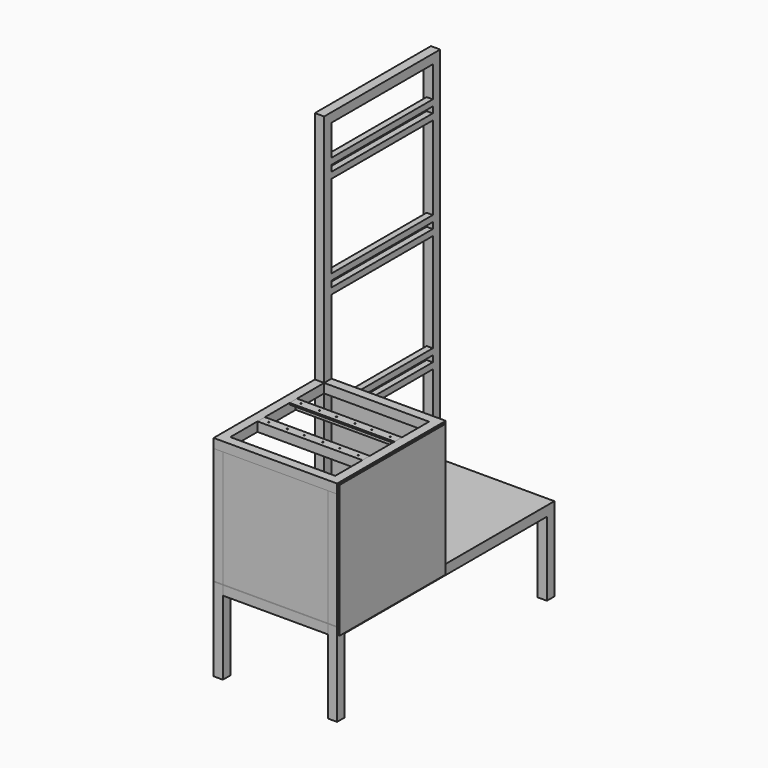
from build123d import *

# Parameters (mm, degrees)
F0_W          = 38.1
F0_H          = 38.1
F1_DEPTH      = 1117.6
F2_W          = 38.1
F2_H          = 38.1
F3_DEPTH      = 304.8
F3_DEPTH_BACK = 558.8
F4_W          = 38.1
F4_H          = 38.1
F5_DEPTH      = 304.8
F5_DEPTH_BACK = 1524
F6_W          = 38.1
F6_H          = 38.1
F7_DEPTH      = 1485.9
F8_W          = 38.1
F8_H          = 38.1
F9_DEPTH      = 431.8
F10_W         = 38.1
F10_H         = 38.1
F11_DEPTH     = 304.8
F12_W         = 38.1
F12_H         = 38.1
F13_DEPTH     = 520.7
F14_W         = 508
F14_H         = 558.8
F14_W_2       = 431.8
F14_H_2       = 482.6
F15_DEPTH     = 38.1
F16_W         = 38.1
F16_H         = 38.1
F17_DEPTH     = 431.8
F18_W         = 38.1
F18_H         = 38.1
F19_DEPTH     = 520.7
F21_DEPTH     = 431.8
F24_W         = 508
F24_H         = 1117.6
F25_DEPTH     = 2.54
F26_W         = 431.8
F26_H         = 482.6
F27_DEPTH     = 1.27
F28_W         = 431.8
F28_H         = 480.06
F29_DEPTH     = 1.27
F30_W         = 546.1
F30_H         = 546.1
F31_DEPTH     = 5.08
F32_W         = 25.4
F32_H         = 25.4
F33_DEPTH     = 520.7
F34_R         = 2.54
F35_DEPTH     = 6.35


with BuildPart() as f1:
    # F0 (on Front) → F1 (new body)
    with BuildSketch(Plane.XZ):
        Rectangle(F0_W, F0_H)
    extrude(amount=F1_DEPTH)

    # F4 (on face) → F5 (join, two sides)
    with BuildSketch(Plane(origin=(0, 0, -19.05), x_dir=(1, 0, 0), z_dir=(0, 0, -1))) as f5_sk:
        with Locations((0, 19.05)):
            Rectangle(F4_W, F4_H)
    extrude(amount=F5_DEPTH)
    extrude(f5_sk.sketch, amount=-F5_DEPTH_BACK)

    # F6 (on face) → F7 (join, through all)
    with BuildSketch(Plane.XY.offset(19.05)):
        with Locations((0, -577.85)):
            Rectangle(F6_W, F6_H)
    extrude(amount=F7_DEPTH)

    # F18 (on face) → F19 (join, through all)
    with BuildSketch(Plane.XZ.offset(38.1)):
        with Locations((0, 1485.9)):
            Rectangle(F18_W, F18_H)
    extrude(amount=F19_DEPTH)

    # F32 (on face) → F33 (join, through all)
    with BuildSketch(Plane(origin=(0, -558.8, 0), x_dir=(-1, 0, 0), z_dir=(0, 1, 0))):
        with Locations((-6.35, 425.45)):
            Rectangle(F32_W, F32_H)
        with Locations((-6.35, 908.05)):
            Rectangle(F32_W, F32_H)
        with Locations((-6.35, 1327.15)):
            Rectangle(F32_W, F32_H)
        with Locations((-6.35, 1276.35)):
            Rectangle(F32_W, F32_H)
        with Locations((-6.35, 857.25)):
            Rectangle(F32_W, F32_H)
        with Locations((-6.35, 374.65)):
            Rectangle(F32_W, F32_H)
    extrude(amount=F33_DEPTH)


with BuildPart() as f1b:
    # F0 (on Front) → F1, piece 2 (new body)
    with BuildSketch(Plane.XZ):
        with Locations((469.9, 0)):
            Rectangle(F0_W, F0_H)
    extrude(amount=F1_DEPTH)

    # F10 (on face) → F11 (join, through all)
    with BuildSketch(Plane(origin=(0, 0, -19.05), x_dir=(1, 0, 0), z_dir=(0, 0, -1))):
        with Locations((469.9, 19.05)):
            Rectangle(F10_W, F10_H)
    extrude(amount=F11_DEPTH)

    # F12 (on face) → F13 (join, through all)
    with BuildSketch(Plane.XY.offset(19.05)):
        with Locations((469.9, -577.85)):
            Rectangle(F12_W, F12_H)
    extrude(amount=F13_DEPTH)


with BuildPart() as f3:
    # F2 (on face) → F3 (new body, two sides)
    with BuildSketch(Plane(origin=(0, 0, -19.05), x_dir=(1, 0, 0), z_dir=(0, 0, -1))) as f3_sk:
        with Locations((469.9, 1098.55)):
            Rectangle(F2_W, F2_H)
    extrude(amount=F3_DEPTH)
    extrude(f3_sk.sketch, amount=-F3_DEPTH_BACK)


with BuildPart() as f3b:
    # F2 (on face) → F3, piece 2 (new body, two sides)
    with BuildSketch(Plane(origin=(0, 0, -19.05), x_dir=(1, 0, 0), z_dir=(0, 0, -1))) as f3_2_sk:
        with Locations((0, 1098.55)):
            Rectangle(F2_W, F2_H)
    extrude(amount=F3_DEPTH)
    extrude(f3_2_sk.sketch, amount=-F3_DEPTH_BACK)


with BuildPart() as f9:
    # F8 (on face) → F9 (new body, through all)
    with BuildSketch(Plane.YZ.offset(19.05)):
        with Locations((-1098.55, 0)):
            Rectangle(F8_W, F8_H)
    extrude(amount=F9_DEPTH)


with BuildPart() as f9b:
    # F8 (on face) → F9, piece 2 (new body, through all)
    with BuildSketch(Plane.YZ.offset(19.05)):
        with Locations((-19.05, 0)):
            Rectangle(F8_W, F8_H)
    extrude(amount=F9_DEPTH)


with BuildPart() as f15:
    # F14 (on face) → F15 (new body)
    with BuildSketch(Plane.XY.offset(539.75)):
        with Locations((234.95, -838.2)):
            Rectangle(F14_W, F14_H)
        with Locations((234.95, -838.2)):
            Rectangle(F14_W_2, F14_H_2, mode=Mode.SUBTRACT)
    extrude(amount=-F15_DEPTH)


with BuildPart() as f17:
    # F16 (on face) → F17 (new body, through all)
    with BuildSketch(Plane.YZ.offset(19.05)):
        with Locations((-577.85, 0)):
            Rectangle(F16_W, F16_H)
    extrude(amount=F17_DEPTH)


with BuildPart() as f21:
    # F20 (on face) → F21 (new body, through all)
    with BuildSketch(Plane.YZ.offset(19.05)):
        Polygon((-736.6, 501.65), (-736.6, 539.75), (-774.7, 539.75), (-774.7, 533.4), (-742.95, 533.4), (-742.95, 501.65), align=None)
    extrude(amount=F21_DEPTH)


with BuildPart() as f21b:
    # F20 (on face) → F21, piece 2 (new body, through all)
    with BuildSketch(Plane.YZ.offset(19.05)):
        Polygon((-901.7, 539.75), (-939.8, 539.75), (-939.8, 501.65), (-933.45, 501.65), (-933.45, 533.4), (-901.7, 533.4), align=None)
    extrude(amount=F21_DEPTH)


with BuildPart() as f25:
    # F24 (on face) → F25 (new body)
    with BuildSketch(Plane.XY.offset(19.05)):
        with Locations((234.95, -558.8)):
            Rectangle(F24_W, F24_H)
    extrude(amount=F25_DEPTH)


with BuildPart() as f27:
    # F26 (on face) → F27 (new body)
    with BuildSketch(Plane(origin=(0, -558.8, 0), x_dir=(-1, 0, 0), z_dir=(0, 1, 0))):
        with Locations((-234.95, 260.35)):
            Rectangle(F26_W, F26_H)
    extrude(amount=-F27_DEPTH)


with BuildPart() as f29:
    # F28 (on face) → F29 (new body)
    with BuildSketch(Plane.XZ.offset(1117.6)):
        with Locations((234.95, 261.62)):
            Rectangle(F28_W, F28_H)
    extrude(amount=-F29_DEPTH)


with BuildPart() as f31:
    # F30 (on face) → F31 (new body)
    with BuildSketch(Plane.YZ.offset(488.95)):
        with Locations((-838.2, 260.35)):
            Rectangle(F30_W, F30_H)
    extrude(amount=F31_DEPTH)


with BuildPart() as f35_tool:
    # F34 (on face) → F35 (new body, through all)
    with BuildSketch(Plane.XY.offset(539.75)):
        with Locations((50.8, -755.65)):
            Circle(F34_R)
        with Locations((127, -755.65)):
            Circle(F34_R)
        with Locations((196.85, -755.65)):
            Circle(F34_R)
        with Locations((273.05, -755.65)):
            Circle(F34_R)
        with Locations((342.9, -755.65)):
            Circle(F34_R)
        with Locations((419.1, -755.65)):
            Circle(F34_R)
        with Locations((50.8, -920.75)):
            Circle(F34_R)
        with Locations((127, -920.75)):
            Circle(F34_R)
        with Locations((196.85, -920.75)):
            Circle(F34_R)
        with Locations((273.05, -920.75)):
            Circle(F34_R)
        with Locations((342.9, -920.75)):
            Circle(F34_R)
        with Locations((419.1, -920.75)):
            Circle(F34_R)
    extrude(amount=-F35_DEPTH)


with BuildPart() as f21_1:
    add(f21.part)

    # F35: cut by f35_tool
    add(f35_tool.part, mode=Mode.SUBTRACT)


with BuildPart() as f21b_1:
    add(f21b.part)

    # F35: cut by f35_tool
    add(f35_tool.part, mode=Mode.SUBTRACT)


solid = Compound([f1.part, f1b.part, f3.part, f3b.part, f9.part, f9b.part, f15.part, f17.part, f25.part, f27.part, f29.part, f31.part, f21_1.part, f21b_1.part])
